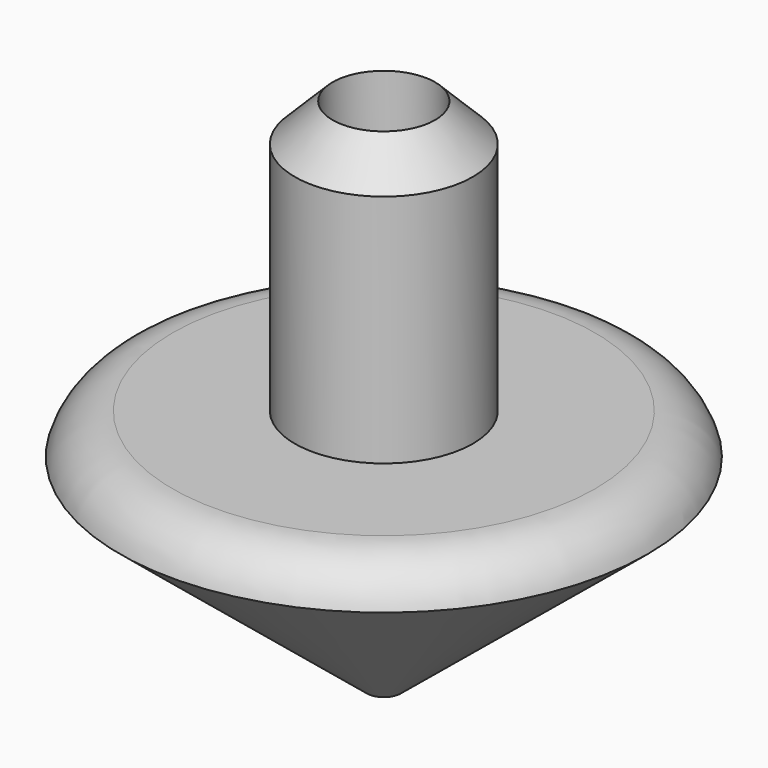
from build123d import *

# Parameters (mm, degrees)
F4_R     = 4.7625
F5_DEPTH = 9.525
F7_R     = 1.5875
F8_DEPTH = 22.225


# Not quite as in the source:
# - a fillet or chamfer that OpenCascade refuses, or shapes differently, is made with other operations: its cross-section is extruded or revolved along the edge and cut away or added


with BuildPart() as f2:
    # F0 (on Front) → F2 (revolve)
    with BuildSketch(Plane.XZ):
        Polygon((0, 50.8), (0, 0), (24.5263007426, 20.1624173125), (24.5263007426, 23.8990907568), (8.2719810307, 23.8990907568), (8.2719810307, 50.8), align=None)
    revolve(axis=Axis((0, 0, 25.4), (0, 0, -1)))

    # F3: fillet of radius 5.08 on 1 edges, made by hand

    # F3_s1 → F3_t2 (revolve, cut)
    with BuildSketch(Plane.XZ):
        with BuildLine():
            ThreePointArc((24.5263007426, 20.1624173125), (22.7079011169, 22.8583047213), (19.6271300205, 23.8990907568))
            Line((19.6271300205, 23.8990907568), (24.5263007426, 23.8990907568))
            Line((24.5263007426, 23.8990907568), (24.5263007426, 20.1624173125))
        make_face()
    revolve(axis=Axis((0, 0, 23.8990907568), (0, 0, -1)), mode=Mode.SUBTRACT)

    # F4 (on face) → F5 (cut)
    with BuildSketch(Plane.XY.offset(50.8)):
        Circle(F4_R)
    extrude(amount=-F5_DEPTH, mode=Mode.SUBTRACT)

    # F6: chamfer of 5.08 on 1 edges, made by hand

    # F6_s1 → F6_t2 (revolve, cut)
    with BuildSketch(Plane.XZ):
        Polygon((8.2719810307, 45.72), (3.1919810307, 50.8), (8.2719810307, 50.8), align=None)
    revolve(axis=Axis((0, 0, 50.8), (0, 0, -1)), mode=Mode.SUBTRACT)

    # F7 (on Top) → F8 (cut)
    with BuildSketch(Plane.XY):
        Circle(F7_R)
    extrude(amount=F8_DEPTH, mode=Mode.SUBTRACT)


solid = f2.part
